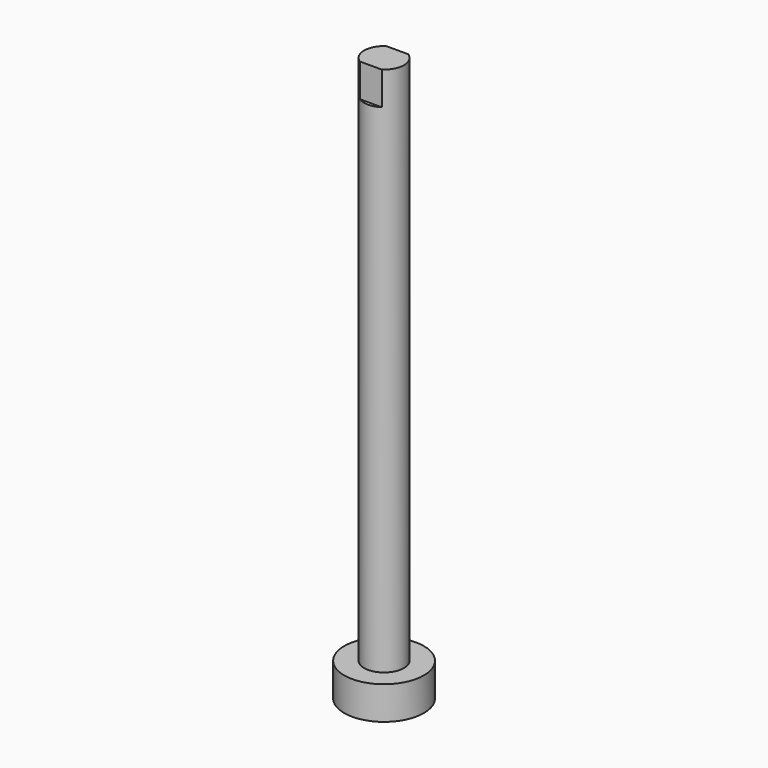
from build123d import *

# Parameters (mm, degrees)
F0_R     = 3
F1_DEPTH = 40
F2_R     = 6
F2_R_2   = 3
F3_DEPTH = 5
F5_DEPTH = 5


with BuildPart() as f1:
    # F0 (on Top) → F1 (new body, symmetric)
    with BuildSketch(Plane.XY):
        Circle(F0_R)
    extrude(amount=F1_DEPTH, both=True)

    # F2 (on face) → F3 (join)
    with BuildSketch(Plane(origin=(0, 0, -40), x_dir=(1, 0, 0), z_dir=(0, 0, -1))):
        Circle(F2_R)
        Circle(F2_R_2, mode=Mode.SUBTRACT)
        Circle(F2_R_2)
    extrude(amount=F3_DEPTH)

    # F4 (on face) → F5 (cut)
    with BuildSketch(Plane.XY.offset(40)):
        with BuildLine():
            Line((4.5341607578, -3.7982849256), (4.5341607578, -2.5))
            Line((4.5341607578, -2.5), (1.6583123952, -2.5))
            ThreePointArc((1.6583123952, -2.5), (0, -3), (-1.6583123952, -2.5))
            Line((-1.6583123952, -2.5), (-4.5341607578, -2.5))
            Line((-4.5341607578, -2.5), (-4.5341607578, -3.7982849256))
            Line((-4.5341607578, -3.7982849256), (4.5341607578, -3.7982849256))
        make_face()
        with BuildLine():
            ThreePointArc((-1.6583123952, -2.5), (0, -3), (1.6583123952, -2.5))
            Line((1.6583123952, -2.5), (-1.6583123952, -2.5))
        make_face()
        with BuildLine():
            Line((1.6583123952, 2.5), (4.5341607578, 2.5))
            Line((4.5341607578, 2.5), (4.5341607578, 3.7982849256))
            Line((4.5341607578, 3.7982849256), (-4.5341607578, 3.7982849256))
            Line((-4.5341607578, 3.7982849256), (-4.5341607578, 2.5))
            Line((-4.5341607578, 2.5), (-1.6583123952, 2.5))
            ThreePointArc((-1.6583123952, 2.5), (0, 3), (1.6583123952, 2.5))
        make_face()
        with BuildLine():
            Line((-1.6583123952, 2.5), (1.6583123952, 2.5))
            ThreePointArc((1.6583123952, 2.5), (0, 3), (-1.6583123952, 2.5))
        make_face()
    extrude(amount=-F5_DEPTH, mode=Mode.SUBTRACT)


solid = f1.part
